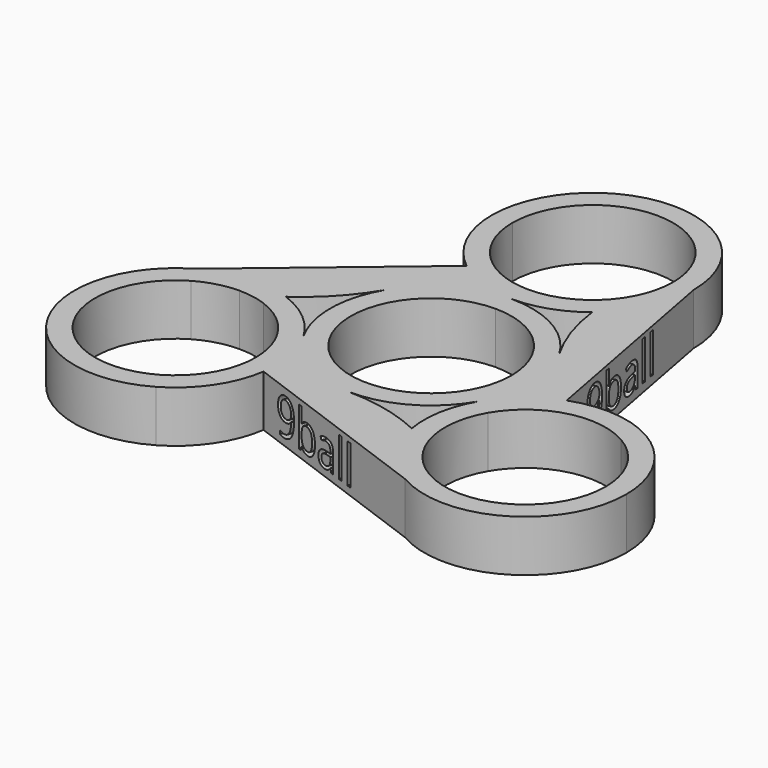
from build123d import *

# Parameters (mm, degrees)
F1_DEPTH     = 7.112
F2_TEXT_SIZE = 7.1615214612
F3_DEPTH     = 2.54
F4_TEXT_SIZE = 7.1211334822
F5_DEPTH     = 2.54
F6_TEXT_SIZE = 7.737324793
F7_DEPTH     = 2.54


# Not quite as in the source:
# - ends of sketch curves that miss each other by under 0.0002 mm in the source are joined
# - a feature names something its author has since deleted; it is built from what else it names
# - Text() gives the source's letters only with a copy of the font that has no kerning and outlines rounded to 1/6400 em; it was checked with that copy


with BuildPart() as f1:
    # F0 (on Top) → F1 (new body)
    with BuildSketch(Plane.XY):
        with BuildLine():
            ThreePointArc((0, 11.1125), (7.8577241059, 7.8577241059), (11.1125, 0))
            ThreePointArc((11.1125, 0), (10.7338507446, -2.8761266387), (9.6237072996, -5.55625))
            Line((9.6237072996, -5.55625), (12.0983748909, -6.985))
            ThreePointArc((12.0983748909, -6.985), (13.4939838315, -3.6157019175), (13.97, 0))
            ThreePointArc((13.97, 0), (13.4755323786, 3.6838739276), (12.0271328398, 7.1069666985))
            ThreePointArc((12.0271328398, 7.1069666985), (6.9237480813, 12.133532565), (-1.95e-08, 13.97))
            Line((-1.95e-08, 13.97), (0, 11.1125))
        make_face()
        with BuildLine():
            ThreePointArc((-9.6237072996, -5.55625), (-9.6237072996, 5.55625), (0, 11.1125))
            Line((0, 11.1125), (0, 13.97))
            ThreePointArc((-1.95e-08, 13.97), (-6.9237478038, 12.1335327234), (-12.0271324949, 7.1069672823))
            ThreePointArc((-12.0271324949, 7.1069672823), (-13.9698214779, 0.0706248839), (-12.0983748909, -6.985))
            Line((-12.0983748909, -6.985), (-9.6237072996, -5.55625))
        make_face()
        with BuildLine():
            Line((12.0983748909, -6.985), (9.6237072996, -5.55625))
            ThreePointArc((9.6237072996, -5.55625), (0, -11.1125), (-9.6237072996, -5.55625))
            Line((-9.6237072996, -5.55625), (-12.0983748909, -6.985))
            ThreePointArc((-12.0983748909, -6.985), (-7.0460734842, -12.0629079602), (-0.1412475033, -13.969285921))
            ThreePointArc((-0.1412475033, -13.969285921), (6.9237481232, -12.1335325411), (12.0983748909, -6.985))
        make_face()
        with BuildLine():
            ThreePointArc((-8.6769039474, 16.9913819188), (-4.593947408, 14.7469507993), (-1.95e-08, 13.97))
            Line((0, 13.97), (0, 16.8275))
            ThreePointArc((0, 16.8275), (-3.65427634, 17.4455290423), (-6.9020826854, 19.2308719809))
            Line((-6.9020826854, 19.2308719809), (-8.6769039474, 16.9913819188))
        make_face()
        with BuildLine():
            ThreePointArc((-12.0271324949, 7.1069672823), (-6.9237478038, 12.1335327234), (-1.95e-08, 13.97))
            ThreePointArc((-1.95e-08, 13.97), (-4.593947408, 14.7469507993), (-8.6769039474, 16.9913819188))
            ThreePointArc((-8.6769039474, 16.9913819188), (-9.8388621787, 11.8752452293), (-12.0271324949, 7.1069672823))
        make_face()
        with BuildLine():
            Line((0, 16.8275), (0, 13.97))
            ThreePointArc((-1.95e-08, 13.97), (4.5939473896, 14.7469507929), (8.6769039474, 16.9913819188))
            ThreePointArc((8.6769039474, 16.9913819188), (12.5773059147, 21.8595168015), (13.97, 27.94))
            Line((13.97, 27.94), (11.1125, 27.94))
            ThreePointArc((11.1125, 27.94), (7.8577241059, 20.0822758941), (0, 16.8275))
        make_face()
        with BuildLine():
            ThreePointArc((19.4187283795, -0.8424940876), (15.2170069875, -3.2683590347), (12.0983750385, -6.9849997443))
            Line((12.0983750385, -6.9849997443), (14.5730424822, -8.41375))
            ThreePointArc((14.5730424822, -8.41375), (21.320623143, -3.2361492554), (29.7529997817, -4.3462927004))
            Line((29.7529997817, -4.3462927004), (31.1817497817, -1.8716251091))
            ThreePointArc((31.1817497817, -1.8716251091), (25.4143155079, -0.0531600677), (19.4187283795, -0.8424940876))
        make_face()
        with BuildLine():
            ThreePointArc((13.97, 0), (13.4939838315, -3.6157019175), (12.0983750385, -6.9849997443))
            ThreePointArc((12.0983750385, -6.9849997443), (15.2170069875, -3.2683590347), (19.4187283795, -0.8424940876))
            ThreePointArc((19.4187283795, -0.8424940876), (15.2933094518, 2.7327644521), (12.0271328398, 7.1069666985))
            ThreePointArc((12.0271328398, 7.1069666985), (13.4755323786, 3.6838739276), (13.97, 0))
        make_face()
        with BuildLine():
            Line((14.5730424822, -8.41375), (12.0983748909, -6.985))
            ThreePointArc((12.0983748909, -6.985), (10.4389854978, -11.5441348126), (10.4389854722, -16.395865042))
            ThreePointArc((10.4389854722, -16.395865042), (12.753195723, -21.9828628158), (17.2117497817, -26.0683748909))
            Line((17.2117497817, -26.0683748909), (18.6404997817, -23.5937072996))
            ThreePointArc((18.6404997817, -23.5937072996), (13.4628990371, -16.8461266387), (14.5730424822, -8.41375))
        make_face()
        with BuildLine():
            ThreePointArc((-10.2267497817, -13.97), (-10.7027659885, -10.3542979399), (-12.0983748909, -6.985))
            Line((-12.0983748909, -6.985), (-14.5730424822, -8.41375))
            ThreePointArc((-14.5730424822, -8.41375), (-13.4628990371, -11.0938733613), (-13.0842497817, -13.97))
            ThreePointArc((-13.0842497817, -13.97), (-14.5730424822, -19.52625), (-18.6404997817, -23.5937072996))
            Line((-18.6404997817, -23.5937072996), (-17.2117497817, -26.0683748909))
            ThreePointArc((-17.2117497817, -26.0683748909), (-12.6422439072, -21.8220248341), (-10.3765164134, -16.010110204))
            ThreePointArc((-10.3765164134, -16.010110204), (-10.2642417492, -14.9928000402), (-10.2267497817, -13.97))
        make_face()
        with BuildLine():
            ThreePointArc((-0.1412475033, -13.969285921), (-7.0460734842, -12.0629079602), (-12.0983748909, -6.985))
            ThreePointArc((-12.0983748909, -6.985), (-10.7027659885, -10.3542979399), (-10.2267497817, -13.97))
            ThreePointArc((-10.2267497817, -13.97), (-10.2642417492, -14.9928000402), (-10.3765164134, -16.010110204))
            ThreePointArc((-10.3765164134, -16.010110204), (-5.36483273, -14.4583271608), (-0.1412475033, -13.969285921))
        make_face()
        with BuildLine():
            Line((-14.5730424822, -8.41375), (-12.0983748909, -6.985))
            ThreePointArc((-12.0983748909, -6.985), (-15.2170068744, -3.2683591296), (-19.4187283795, -0.8424940876))
            Line((-19.4187283795, -0.8424940876), (-20.396050939, -3.5276657515))
            ThreePointArc((-20.396050939, -3.5276657515), (-17.0537724691, -5.4573311258), (-14.5730424822, -8.41375))
        make_face()
        with BuildLine():
            ThreePointArc((8.6769039474, 16.9913819188), (9.8388622875, 11.8752449082), (12.0271328398, 7.1069666985))
            ThreePointArc((12.0271328398, 7.1069666985), (15.2933094518, 2.7327644521), (19.4187283795, -0.8424940876))
            Line((19.4187283795, -0.8424940876), (13.97, 27.94))
            ThreePointArc((13.97, 27.94), (12.5773059147, 21.8595168015), (8.6769039474, 16.9913819188))
        make_face()
        with BuildLine():
            ThreePointArc((-19.4187283795, -0.8424940876), (-15.293309221, 2.7327647003), (-12.0271324949, 7.1069672823))
            ThreePointArc((-12.0271324949, 7.1069672823), (-9.8388621787, 11.8752452293), (-8.6769039474, 16.9913819188))
            Line((-8.6769039474, 16.9913819188), (-31.1817497817, -1.8716251091))
            ThreePointArc((-31.1817497817, -1.8716251091), (-27.8124518418, -0.4760162067), (-24.1967497817, 0))
            ThreePointArc((-24.1967497817, 0), (-21.7708847397, -0.2122356904), (-19.4187283795, -0.8424940876))
        make_face()
        with BuildLine():
            ThreePointArc((-13.97, 27.94), (-12.5773059147, 21.8595168015), (-8.6769039474, 16.9913819188))
            Line((-8.6769039474, 16.9913819188), (-6.9020826854, 19.2308719809))
            ThreePointArc((-6.9020826854, 19.2308719809), (-10.0046751594, 23.1032520012), (-11.1125, 27.94))
            Line((-11.1125, 27.94), (-13.97, 27.94))
        make_face()
        with BuildLine():
            ThreePointArc((10.4389854722, -16.395865042), (5.2800111814, -14.6107766948), (-0.1412475033, -13.969285921))
            ThreePointArc((-0.1412475033, -13.969285921), (-5.36483273, -14.4583271608), (-10.3765164134, -16.010110204))
            Line((-10.3765164134, -16.010110204), (17.2117497817, -26.0683748909))
            ThreePointArc((17.2117497817, -26.0683748909), (12.753195723, -21.9828628158), (10.4389854722, -16.395865042))
        make_face()
        with BuildLine():
            Line((-20.396050939, -3.5276657515), (-19.4187283795, -0.8424940876))
            ThreePointArc((-19.4187283795, -0.8424940876), (-21.7708847397, -0.2122356904), (-24.1967497817, 0))
            Line((-24.1967497817, 0), (-24.1967497817, -2.8575))
            ThreePointArc((-24.1967497817, -2.8575), (-22.2670844074, -3.0263238447), (-20.396050939, -3.5276657515))
        make_face()
        with BuildLine():
            ThreePointArc((-11.1125, 27.94), (0, 39.0525), (11.1125, 27.94))
            Line((11.1125, 27.94), (13.97, 27.94))
            ThreePointArc((13.97, 27.94), (0, 41.91), (-13.97, 27.94))
            Line((-13.97, 27.94), (-11.1125, 27.94))
        make_face()
        with BuildLine():
            Line((-29.7529997817, -4.3462927004), (-31.1817497817, -1.8716251091))
            ThreePointArc((-31.1817497817, -1.8716251091), (-36.2951246726, -20.955), (-17.2117497817, -26.0683748909))
            Line((-17.2117497817, -26.0683748909), (-18.6404997817, -23.5937072996))
            ThreePointArc((-18.6404997817, -23.5937072996), (-33.8204570813, -19.52625), (-29.7529997817, -4.3462927004))
        make_face()
        with BuildLine():
            ThreePointArc((-24.1967497817, 0), (-27.8124518418, -0.4760162067), (-31.1817497817, -1.8716251091))
            Line((-31.1817497817, -1.8716251091), (-29.7529997817, -4.3462927004))
            ThreePointArc((-29.7529997817, -4.3462927004), (-27.0728764204, -3.2361492554), (-24.1967497817, -2.8575))
            Line((-24.1967497817, -2.8575), (-24.1967497817, 0))
        make_face()
        with BuildLine():
            Line((31.1817497817, -1.8716251091), (29.7529997817, -4.3462927004))
            ThreePointArc((29.7529997817, -4.3462927004), (33.8204570813, -8.41375), (35.3092497817, -13.97))
            ThreePointArc((35.3092497817, -13.97), (29.7529997817, -23.5937072996), (18.6404997817, -23.5937072996))
            Line((18.6404997817, -23.5937072996), (17.2117497817, -26.0683748909))
            ThreePointArc((17.2117497817, -26.0683748909), (31.1817497817, -26.0683748909), (38.1667497817, -13.97))
            ThreePointArc((38.1667497817, -13.97), (36.2951246726, -6.985), (31.1817497817, -1.8716251091))
        make_face()
    extrude(amount=F1_DEPTH)

    # F2 (on face) → F3 (cut)
    with BuildSketch(Plane(origin=(18.5929210217, 3.5197705981, 0), x_dir=(-0.1860034472, 0.9825490917, 0), z_dir=(0.9825490917, 0.1860034472, 0))):
        with Locations((0, 1.1036787951)):
            Text('9ball', F2_TEXT_SIZE, font='Open Sans', text_align=(TextAlign.LEFT, TextAlign.BOTTOM))
    extrude(amount=-F3_DEPTH, mode=Mode.SUBTRACT)

    # F4 (on face) → F5 (cut)
    with BuildSketch(Plane(origin=(-6.3696458707, -17.4709546152, 0), x_dir=(0.9395068895, -0.3425300054, 0), z_dir=(-0.3425300054, -0.9395068895, 0))):
        with Locations((-1.6083233058, 0.9911322268)):
            Text('9ball', F4_TEXT_SIZE, font='Open Sans', text_align=(TextAlign.LEFT, TextAlign.BOTTOM))
    extrude(amount=-F5_DEPTH, mode=Mode.SUBTRACT)

    # F6 (on face) → F7 (cut)
    with BuildSketch(Plane(origin=(-11.9454675897, 14.2517524448, 0), x_dir=(-0.766393131, -0.6423718306, 0), z_dir=(-0.6423718306, 0.766393131, 0))):
        with Locations((0.6862082519, 0.7770366501)):
            Text('9ball', F6_TEXT_SIZE, font='Open Sans', text_align=(TextAlign.LEFT, TextAlign.BOTTOM))
    extrude(amount=-F7_DEPTH, mode=Mode.SUBTRACT)


solid = f1.part
